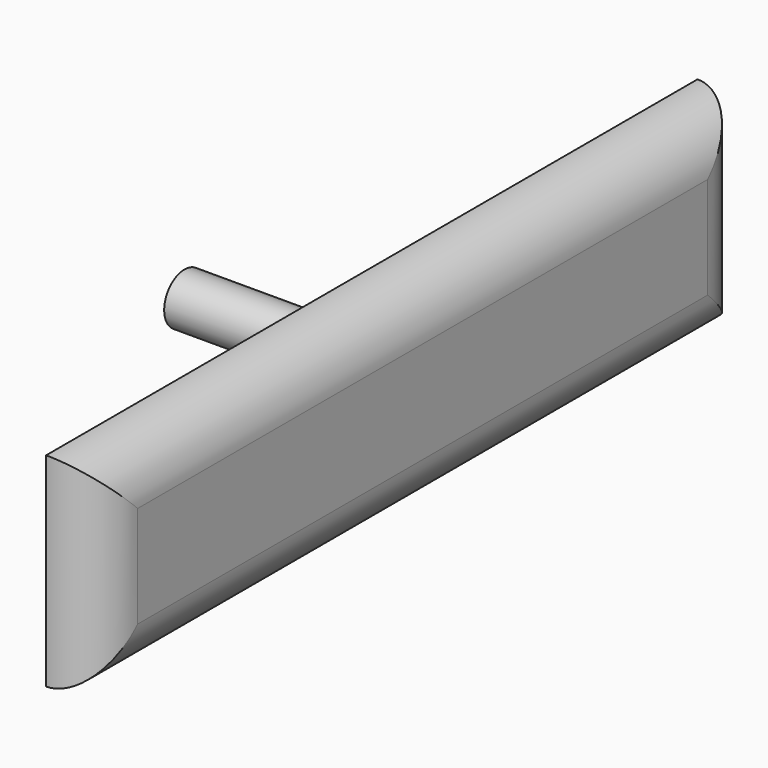
from build123d import *

# Parameters (mm, degrees)
F0_W          = 1.27
F0_H          = 20.32
F1_DEPTH      = 2.54
F1_DEPTH_BACK = 2.54
F2_R          = 1.26999
F3_R          = 0.635
F4_DEPTH      = 5.08


# Not quite as in the source:
# - a fillet or chamfer is up to 0.001 mm smaller than in the source, because OpenCascade refuses the exact size


with BuildPart() as f1:
    # F0 (on Top) → F1 (new body, two sides)
    with BuildSketch(Plane.XY) as f1_sk:
        with Locations((0.635, -0.508000601)):
            Rectangle(F0_W, F0_H)
    extrude(amount=F1_DEPTH)
    extrude(f1_sk.sketch, amount=-F1_DEPTH_BACK)

    # F2 (radius 1.27 in the source; OpenCascade refuses exactly that, so slightly less here)
    f2_edges = [f1.edges().sort_by_distance(p)[0] for p in [
        (1.27, 9.651999, 0),
        (1.27, -0.508001, 2.54),
        (1.27, -0.508001, -2.54),
        (1.27, -10.668001, 0),
    ]]
    fillet(f2_edges, radius=F2_R)

    # F3 (on face) → F4 (join)
    with BuildSketch(Plane(origin=(0, 0, 0), x_dir=(0, -1, 0), z_dir=(-1, 0, 0))):
        Circle(F3_R)
    extrude(amount=F4_DEPTH)


solid = f1.part
